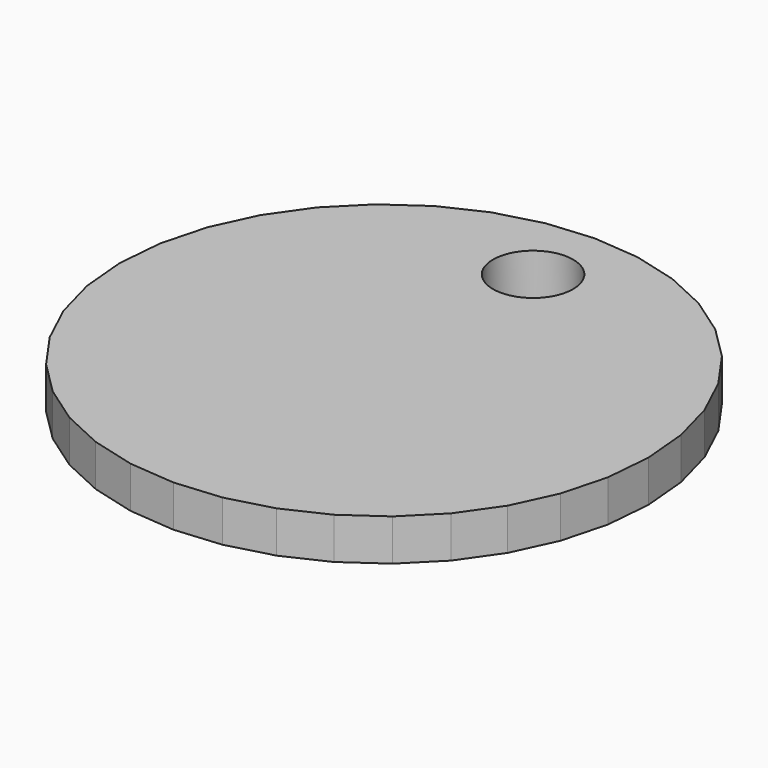
from build123d import *

# Parameters (mm, degrees)
F1_DEPTH = 6.35
F4_R     = 6.1144864015
F5_DEPTH = 6.351


# Not quite as in the source:
# - the program builds the solid bodies; features that only make, move or delete a surface that nothing else refers to are left out


with BuildPart() as f1:
    # F0 (on Top) → F1 (new body)
    with BuildSketch(Plane.XY):
        Polygon((37.8358727575, 13.8656235676), (34.8533205688, 20.2251039445), (30.8117678713, 25.9700547725), (25.8340151985, 30.9259186276), (20.0713090466, 34.9421140946), (13.6987463258, 37.8966111063), (6.9099541298, 39.6996387661), (-0.0887935258, 40.2964129911), (-7.084843235, 39.6688010983), (-13.8656235676, 37.8358727575), (-20.2251039445, 34.8533205688), (-25.9700547725, 30.8117678713), (-30.9259186276, 25.8340151985), (-34.9421140946, 20.0713090466), (-37.8966111063, 13.6987463258), (-39.6996387661, 6.9099541298), (-40.2964129911, -0.0887935258), (-39.6688010983, -7.084843235), (-37.8358727575, -13.8656235676), (-34.8533205688, -20.2251039445), (-30.8117678713, -25.9700547725), (-25.8340151985, -30.9259186276), (-20.0713090466, -34.9421140946), (-13.6987463258, -37.8966111063), (-6.9099541298, -39.6996387661), (0.0887935258, -40.2964129911), (7.084843235, -39.6688010983), (13.8656235676, -37.8358727575), (20.2251039445, -34.8533205688), (25.9700547725, -30.8117678713), (30.9259186276, -25.8340151985), (34.9421140946, -20.0713090466), (37.8966111063, -13.6987463258), (39.6996387661, -6.9099541298), (40.2964129911, 0.0887935258), (39.6688010983, 7.084843235), align=None)
    extrude(amount=F1_DEPTH)

    # F4 (on face) → F5 (cut, through all)
    with BuildSketch(Plane.XY.offset(6.35)):
        with Locations((0, 28.4479867001)):
            Circle(F4_R)
    extrude(amount=-F5_DEPTH, mode=Mode.SUBTRACT)


solid = f1.part
